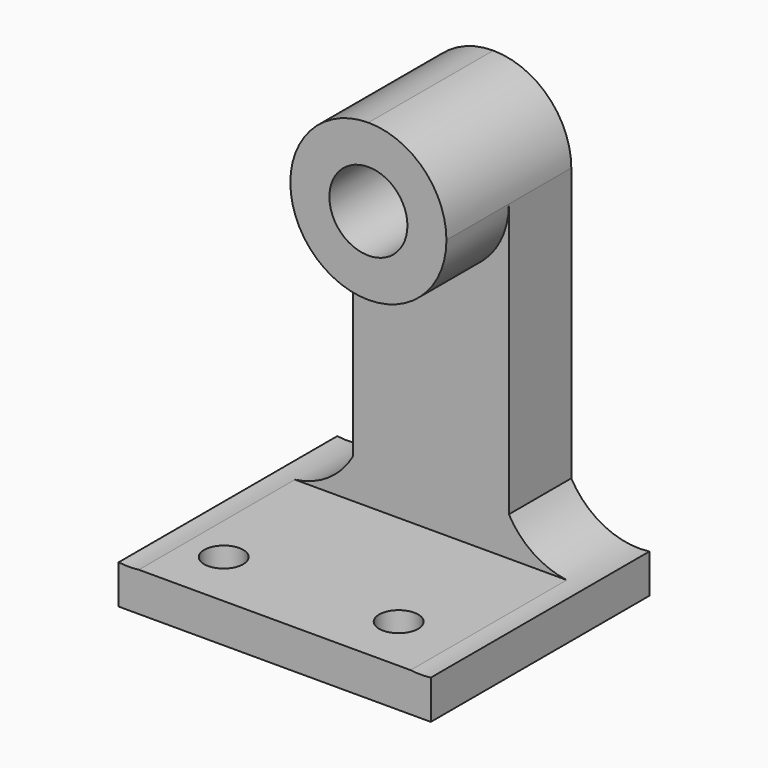
from build123d import *

# Parameters (mm, degrees)
F1_DEPTH = 50.8
F3_DEPTH = 12.7
F5_R     = 3.175
F6_DEPTH = 6.351
F8_DEPTH = 6.351
F9_DEPTH = 44.451


with BuildPart() as f1:
    # F0 (on Right) → F1 (new body)
    with BuildSketch(Plane.YZ):
        Polygon((-44.45, 0), (0, 0), (0, 69.85), (-12.7, 69.85), (-12.7, 6.35), (-44.45, 6.35), align=None)
    extrude(amount=F1_DEPTH)

    # F2 (on face) → F3 (join)
    with BuildSketch(Plane.XZ.offset(12.7)):
        with BuildLine():
            ThreePointArc((38.1, 57.15), (34.3802561211, 66.1302561211), (25.4, 69.85))
            ThreePointArc((25.4, 69.85), (16.4197438789, 48.1697438789), (38.1, 57.15))
        make_face()
        with BuildLine():
            ThreePointArc((31.75, 57.15), (20.9098719395, 52.6598719395), (25.4, 63.5))
            ThreePointArc((25.4, 63.5), (29.8901280605, 61.6401280605), (31.75, 57.15))
        make_face(mode=Mode.SUBTRACT)
    extrude(amount=F3_DEPTH)

    # F5 (on face) → F6 (cut, through all)
    with BuildSketch(Plane.XY.offset(6.35)):
        with BuildLine():
            ThreePointArc((12.7, -34.9846648967), (9.525, -31.8096648967), (6.35, -34.9846648967))
            ThreePointArc((6.35, -34.9846648967), (9.525, -38.1596648967), (12.7, -34.9846648967))
        make_face()
        with Locations((37.9935720786, -34.9846648967)):
            Circle(F5_R)
    extrude(amount=-F6_DEPTH, mode=Mode.SUBTRACT)

    # F7 (on face) → F8 (cut, through all)
    with BuildSketch(Plane.XY.offset(6.35)):
        with BuildLine():
            Line((9.525, -38.1596648967), (9.525, -34.9846648967))
            Line((9.525, -34.9846648967), (6.35, -34.9846648967))
            ThreePointArc((6.35, -34.9846648967), (7.2799359697, -37.229728927), (9.525, -38.1596648967))
        make_face()
    extrude(amount=-F8_DEPTH, mode=Mode.SUBTRACT)

    # F4 (on face) → F9 (cut, through all)
    with BuildSketch(Plane(origin=(0, 0, 0), x_dir=(-1, 0, 0), z_dir=(0, 1, 0))):
        with BuildLine():
            ThreePointArc((-50.8, 6.35), (-43.4796733765, 7.5843467529), (-38.1, 12.7))
            Line((-38.1, 12.7), (-50.8, 12.7))
            Line((-50.8, 12.7), (-50.8, 6.35))
        make_face()
        with BuildLine():
            ThreePointArc((-38.1, 57.15), (-34.3802561211, 66.1302561211), (-25.4, 69.85))
            Line((-25.4, 69.85), (-50.8, 69.85))
            Line((-50.8, 69.85), (-50.8, 12.7))
            Line((-50.8, 12.7), (-38.1, 12.7))
            Line((-38.1, 12.7), (-38.1, 57.15))
        make_face()
        with BuildLine():
            Line((0, 69.85), (-25.4, 69.85))
            ThreePointArc((-25.4, 69.85), (-16.4197438789, 66.1302561211), (-12.7, 57.15))
            Line((-12.7, 57.15), (-12.7, 12.7))
            ThreePointArc((-12.7, 12.7), (-7.3203266235, 7.5843467529), (0, 6.35))
            Line((0, 6.35), (0, 69.85))
        make_face()
        with BuildLine():
            ThreePointArc((-19.05, 57.15), (-20.9098719395, 61.6401280605), (-25.4, 63.5))
            ThreePointArc((-25.4, 63.5), (-29.8901280605, 52.6598719395), (-19.05, 57.15))
        make_face()
    extrude(amount=-F9_DEPTH, mode=Mode.SUBTRACT)


solid = f1.part
